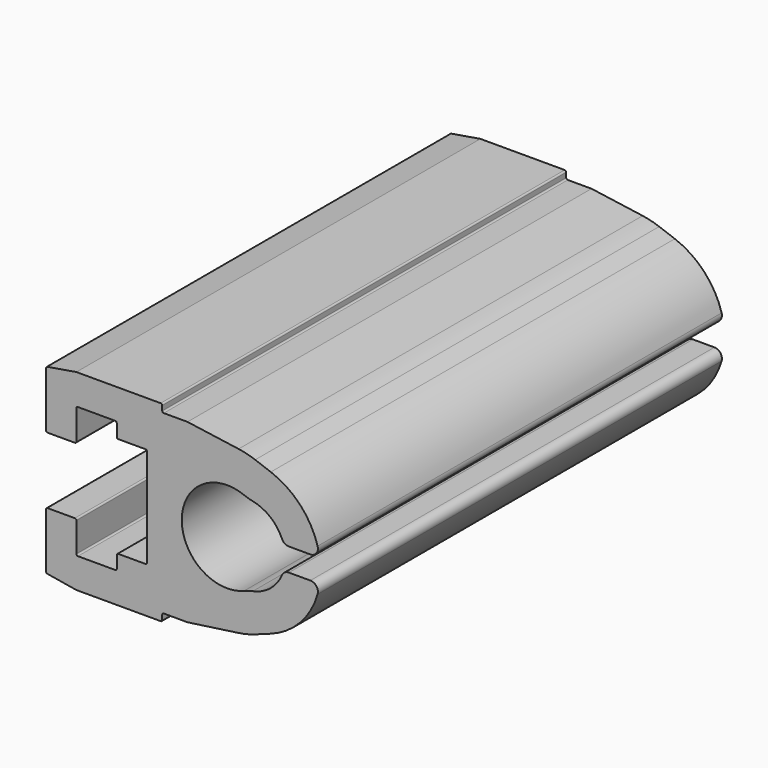
from build123d import *

# Parameters (mm, degrees)
F1_DEPTH = 50


# Not quite as in the source:
# - ends of sketch curves that miss each other by under 0.0002 mm in the source are joined


with BuildPart() as f1:
    # F0 (on Front) → F1 (new body, symmetric)
    with BuildSketch(Plane.XZ):
        with BuildLine():
            Line((53.992555, -15.220268), (57.083133, -14.095389))
            ThreePointArc((57.083133, -14.095389), (62.9018568836, -10.252747544), (66.3544503107, -4.1944440905))
            ThreePointArc((66.3544503107, -4.1944440905), (66.1141142416, -2.8747683688), (64.914288, -2.275))
            Line((64.914288, -2.275), (60.670593, -2.275))
            ThreePointArc((60.670593, -2.275), (59.8472095147, -2.5211899521), (59.2941043505, -3.1789471518))
            ThreePointArc((59.2941043505, -3.1789471518), (56.9827494729, -6.2209259886), (53.52425904, -7.8441451998))
            ThreePointArc((53.52425904, -7.8441451998), (52.6431740995, -8.0626756758), (51.7855370008, -8.3602070021))
            ThreePointArc((51.7855370008, -8.3602070021), (39.452831, 0), (51.7855371982, 8.3602074972))
            ThreePointArc((51.7855371982, 8.3602074972), (52.6431743712, 8.0626765952), (53.524259133, 7.844145664))
            ThreePointArc((53.524259133, 7.844145664), (56.9827494729, 6.2209259886), (59.2941043849, 3.1789471667))
            ThreePointArc((59.2941043849, 3.1789471667), (59.8472095147, 2.5211899521), (60.670593, 2.275))
            Line((60.670593, 2.275), (64.914288, 2.275))
            ThreePointArc((64.914288, 2.275), (66.1141145297, 2.8747687527), (66.3544497778, 4.1944449353))
            ThreePointArc((66.3544497778, 4.1944449353), (62.9018565554, 10.2527478944), (57.0831331177, 14.0953893235))
            Line((57.0831331177, 14.0953893235), (53.992555, 15.220268))
            ThreePointArc((53.992555, 15.220268), (52.3736165632, 15.715360306), (50.7118440801, 16.0387645685))
            Line((50.7118440801, 16.0387645685), (40.585713, 17.465))
            Line((40.585713, 17.465), (35.885713, 17.465))
            ThreePointArc((35.885713, 17.465), (35.6735809656, 17.5528679656), (35.585713, 17.765))
            Line((35.585713, 17.765), (35.585713, 18.7))
            ThreePointArc((35.585713, 18.7), (35.4978450344, 18.9121320344), (35.285713, 19))
            Line((35.285713, 19), (18.585713, 19))
            Line((18.585713, 19), (12.836393, 18.04178))
            ThreePointArc((12.836393, 18.04178), (12.656806899, 17.9397743434), (12.585713, 17.745862))
            Line((12.585713, 17.745862), (12.585713, 6.875))
            ThreePointArc((12.585713, 6.875), (12.6735809656, 6.6628679656), (12.885713, 6.575))
            Line((12.885713, 6.575), (18.285713, 6.575))
            ThreePointArc((18.285713, 6.575), (18.4978450344, 6.6628679656), (18.585713, 6.875))
            Line((18.585713, 6.875), (18.585713, 12.7))
            ThreePointArc((18.585713, 12.7), (18.6735809656, 12.9121320344), (18.885713, 13))
            Line((18.885713, 13), (26.285713, 13))
            ThreePointArc((26.285713, 13), (26.4978450344, 12.9121320344), (26.585713, 12.7))
            Line((26.585713, 12.7), (26.585713, 10.3))
            ThreePointArc((26.585713, 10.3), (26.6735809656, 10.0878679656), (26.885713, 10))
            Line((26.885713, 10), (32.285713, 10))
            ThreePointArc((32.285713, 10), (32.4978450344, 9.9121320344), (32.585713, 9.7))
            Line((32.585713, 9.7), (32.585713, -9.7))
            ThreePointArc((32.585713, -9.7), (32.4978450344, -9.9121320344), (32.285713, -10))
            Line((32.285713, -10), (26.885713, -10))
            ThreePointArc((26.885713, -10), (26.6735809656, -10.0878679656), (26.585713, -10.3))
            Line((26.585713, -10.3), (26.585713, -12.7))
            ThreePointArc((26.585713, -12.7), (26.4978450344, -12.9121320344), (26.285713, -13))
            Line((26.285713, -13), (18.885713, -13))
            ThreePointArc((18.885713, -13), (18.6735809656, -12.9121320344), (18.585713, -12.7))
            Line((18.585713, -12.7), (18.585713, -6.875))
            ThreePointArc((18.585713, -6.875), (18.4978450344, -6.6628679656), (18.285713, -6.575))
            Line((18.285713, -6.575), (12.885713, -6.575))
            ThreePointArc((12.885713, -6.575), (12.6735809656, -6.6628679656), (12.585713, -6.875))
            Line((12.585713, -6.875), (12.585713, -17.745862))
            ThreePointArc((12.585713, -17.745862), (12.656806899, -17.9397743434), (12.8363929795, -18.0417801231))
            Line((12.8363929795, -18.0417801231), (18.585713, -19))
            Line((18.585713, -19), (35.285713, -19))
            ThreePointArc((35.285713, -19), (35.4978450344, -18.9121320344), (35.585713, -18.7))
            Line((35.585713, -18.7), (35.585713, -17.765))
            ThreePointArc((35.585713, -17.765), (35.6735809656, -17.5528679656), (35.885713, -17.465))
            Line((35.885713, -17.465), (40.585713, -17.465))
            Line((40.585713, -17.465), (50.711844, -16.038764))
            ThreePointArc((50.711844, -16.038764), (52.3736165632, -15.715360306), (53.992555, -15.220268))
        make_face()
    extrude(amount=F1_DEPTH, both=True)


solid = f1.part
